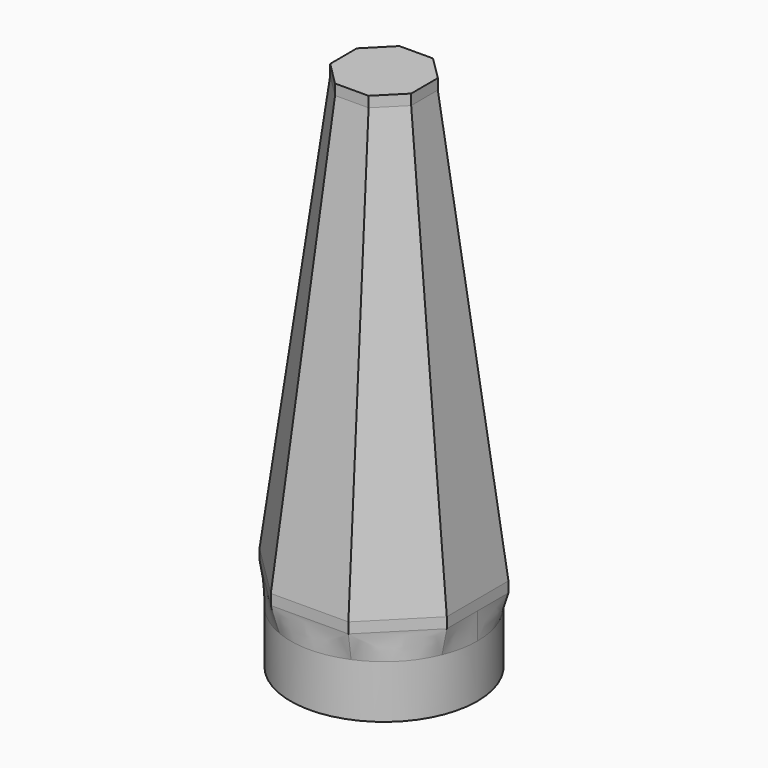
from build123d import *

# Parameters (mm, degrees)
F0_R      = 17.625
F1_DEPTH  = 10
F3_START  = 5
F3_DEPTH  = 2
F6_DEPTH  = 2
F1_FACE_R = 17.625


# Not quite as in the source:
# - a feature names something its author has since deleted; it is built from what else it names


with BuildPart() as f1:
    # F0 (on Top) → F1 (new body)
    with BuildSketch(Plane.XY):
        Circle(F0_R)
    extrude(amount=F1_DEPTH)



with BuildPart() as f3:
    # F2 (on face) → F3 (new body)
    with BuildSketch(Plane.XY.offset(10).offset(F3_START)):
        Polygon((7.3588174532, -17.6007367997), (17.6490700676, -7.2421306223), (17.6007367997, 7.3588174532), (7.2421306223, 17.6490700676), (-7.3588174532, 17.6007367997), (-17.6490700676, 7.2421306223), (-17.6007367997, -7.3588174532), (-7.2421306223, -17.6490700676), align=None)
    extrude(amount=F3_DEPTH)



with BuildPart() as f6:
    # F5 (on offset) → F6 (new body)
    with BuildSketch(Plane.XY.offset(97)):
        Polygon((-7.6354132917, 3.1331203401), (-7.6145031545, -3.1836018769), (-3.1331203401, -7.6354132917), (3.1836018769, -7.6145031545), (7.6354132917, -3.1331203401), (7.6145031545, 3.1836018769), (3.1331203401, 7.6354132917), (-3.1836018769, 7.6145031545), align=None)
    extrude(amount=F6_DEPTH)


with BuildPart() as f3_1:
    add(f3.part)

    add(f6.part)  # F7 merges F6
    # F3_face (on face) → F7 section 0
    with BuildSketch(Plane.XY.offset(17)):
        Polygon((-17.6007367997, -7.3588174532), (-7.2421306223, -17.6490700676), (7.3588174532, -17.6007367997), (17.6490700676, -7.2421306223), (17.6007367997, 7.3588174532), (7.2421306223, 17.6490700676), (-7.3588174532, 17.6007367997), (-17.6490700676, 7.2421306223), align=None)
    # F6_face (on face) → F7 section 1
    with BuildSketch(Plane(origin=(0, 0, 97), x_dir=(1, 0, 0), z_dir=(0, 0, -1))):
        Polygon((-3.1836018769, -7.6145031545), (3.1331203401, -7.6354132917), (7.6145031545, -3.1836018769), (7.6354132917, 3.1331203401), (3.1836018769, 7.6145031545), (-3.1331203401, 7.6354132917), (-7.6145031545, 3.1836018769), (-7.6354132917, -3.1331203401), align=None)
    loft()


with BuildPart() as f1_1:
    add(f1.part)

    add(f3_1.part)  # F8 merges F3
    # F3_face1 (on face) → F8 section 0
    with BuildSketch(Plane(origin=(0, 0, 15), x_dir=(1, 0, 0), z_dir=(0, 0, -1))):
        Polygon((-7.2421306223, 17.6490700676), (-17.6007367997, 7.3588174532), (-17.6490700676, -7.2421306223), (-7.3588174532, -17.6007367997), (7.2421306223, -17.6490700676), (17.6007367997, -7.3588174532), (17.6490700676, 7.2421306223), (7.3588174532, 17.6007367997), align=None)
    # F1_face (on face) → F8 section 1
    with BuildSketch(Plane.XY.offset(10)):
        Circle(F1_FACE_R)
    loft()


solid = f1_1.part
